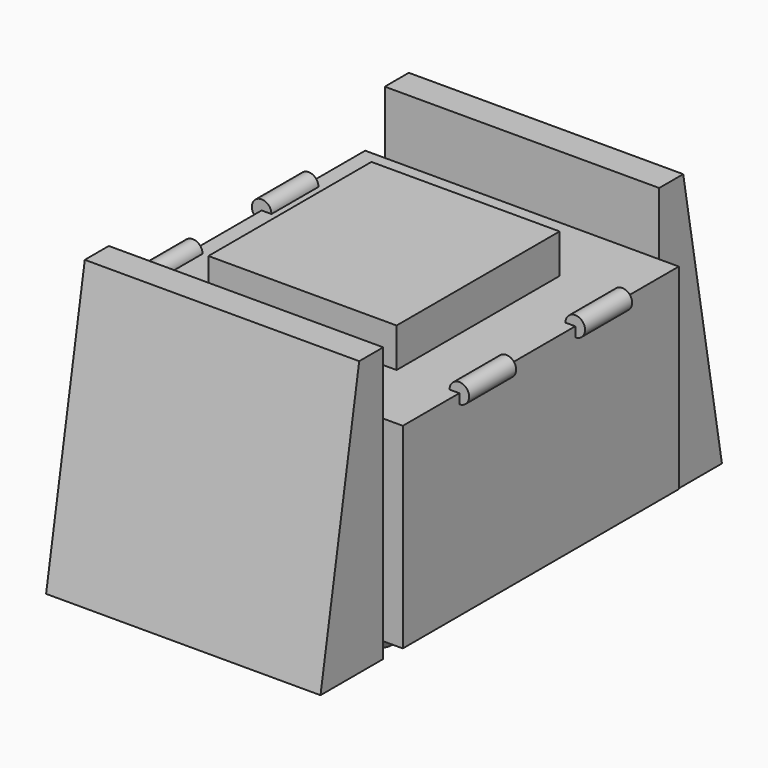
from build123d import *

# Parameters (mm, degrees)
F0_W        = 121.92
F0_H        = 25.4
F1_DEPTH    = 66.0019
F2_W        = 203.2
F2_H        = 223.52
F3_DEPTH    = 25.4
F2_W_2      = 121.92
F2_H_2      = 132.0038
F4_DEPTH    = 127
F5_W        = 127
F5_H        = 177.8
F6_DEPTH    = 38.1
F7_R        = 38.09999
F8_T1_DEPTH = 299.2776586204
F9_W        = 177.8
F9_H        = 177.8
F10_DEPTH   = 50.8
F11_SIZE2   = 31.350927
F11_SIZE    = 177.79999
F12_W       = 177.8
F12_H       = 177.8
F13_DEPTH   = 50.8
F14_SIZE2   = 31.350927
F14_SIZE    = 177.79999
F15_R       = 6.35
F16_DEPTH   = 38.1
F17_R       = 6.35
F18_DEPTH   = 38.1
F19_R       = 6.35
F20_DEPTH   = 38.1
F21_R       = 6.35
F22_DEPTH   = 38.1


# Not quite as in the source:
# - a fillet or chamfer that OpenCascade refuses, or shapes differently, is made with other operations: its cross-section is extruded or revolved along the edge and cut away or added
# - a fillet or chamfer is up to 0.001 mm smaller than in the source, because OpenCascade refuses the exact size


with BuildPart() as f1:
    # F0 (on Front) → F1 (new body, symmetric)
    with BuildSketch(Plane.XZ):
        Rectangle(F0_W, F0_H)
    extrude(amount=F1_DEPTH, both=True)

    # F2 (on face) → F3 (join)
    with BuildSketch(Plane(origin=(0, 0, -12.7), x_dir=(1, 0, 0), z_dir=(0, 0, -1))):
        Rectangle(F2_W, F2_H)
    extrude(amount=F3_DEPTH)

    # F2 (on face) → F4 (join)
    with BuildSketch(Plane(origin=(0, 0, -12.7), x_dir=(1, 0, 0), z_dir=(0, 0, -1))):
        Rectangle(F2_W, F2_H)
        Rectangle(F2_W_2, F2_H_2, mode=Mode.SUBTRACT)
        Rectangle(F2_W_2, F2_H_2)
    extrude(amount=F4_DEPTH)

    # F5 (on face) → F6 (join)
    with BuildSketch(Plane(origin=(0, 0, -139.7), x_dir=(1, 0, 0), z_dir=(0, 0, -1))):
        Rectangle(F5_W, F5_H)
    extrude(amount=F6_DEPTH)

    # F7 (radius 38.1 in the source; OpenCascade refuses exactly that, so slightly less here)
    f7_edges = [f1.edges().sort_by_distance(p)[0] for p in [
        (0, -88.9, -177.8),
        (0, 88.9, -177.8),
    ]]
    fillet(f7_edges, radius=F7_R)

    # F8: chamfer of 38.1 x 13.8672659255 on 2 edges, made by hand

    # F8_s2 → F8_t1 (cut)
    with BuildSketch(Plane.XZ.offset(-149.6388293102)):
        Polygon((63.5, -139.7), (49.6327340745, -177.8), (63.5, -177.8), align=None)
        Polygon((-49.6327340745, -177.8), (-63.5, -139.7), (-63.5, -177.8), align=None)
    extrude(amount=F8_T1_DEPTH, mode=Mode.SUBTRACT)

    # F9 (on face) → F10 (join)
    with BuildSketch(Plane.XZ.offset(111.76)):
        with Locations((1.431e-07, -60.9599946499)):
            Rectangle(F9_W, F9_H)
    extrude(amount=F10_DEPTH)

    # F11 (size 177.8 and 31.35093717 in the source; OpenCascade refuses exactly that, so slightly less here)
    f11_edges = [f1.edges().sort_by_distance(p)[0] for p in [
        (0, -162.56, 27.940005),
    ]]
    f11_side = f1.faces().sort_by_distance((0, -162.56, -60.959995))[0]
    chamfer(f11_edges, length=F11_SIZE, length2=F11_SIZE2, reference=f11_side)

    # F12 (on face) → F13 (join)
    with BuildSketch(Plane(origin=(0, 111.76, 0), x_dir=(-1, 0, 0), z_dir=(0, 1, 0))):
        with Locations((0.0031362507, -60.9484007582)):
            Rectangle(F12_W, F12_H)
    extrude(amount=F13_DEPTH)

    # F14 (size 177.8 and 31.35093717 in the source; OpenCascade refuses exactly that, so slightly less here)
    f14_edges = [f1.edges().sort_by_distance(p)[0] for p in [
        (-0.003136, 162.56, 27.951599),
    ]]
    f14_side = f1.faces().sort_by_distance((-0.003136, 162.56, -60.948401))[0]
    chamfer(f14_edges, length=F14_SIZE, length2=F14_SIZE2, reference=f14_side)

    # F15 (on face) → F16 (join)
    with BuildSketch(Plane(origin=(0, 66.0019, 0), x_dir=(-1, 0, 0), z_dir=(0, 1, 0))):
        with Locations((101.6, -12.7)):
            Circle(F15_R)
    extrude(amount=-F16_DEPTH)

    # F17 (on face) → F18 (join)
    with BuildSketch(Plane.XZ.offset(66.0019)):
        with Locations((-101.6, -12.7)):
            Circle(F17_R)
    extrude(amount=-F18_DEPTH)

    # F19 (on face) → F20 (join)
    with BuildSketch(Plane.XZ.offset(66.0019)):
        with Locations((101.6, -12.7)):
            Circle(F19_R)
    extrude(amount=-F20_DEPTH)

    # F21 (on face) → F22 (join)
    with BuildSketch(Plane(origin=(0, 66.0019, 0), x_dir=(-1, 0, 0), z_dir=(0, 1, 0))):
        with Locations((-101.6, -12.7)):
            Circle(F21_R)
    extrude(amount=-F22_DEPTH)


solid = f1.part
